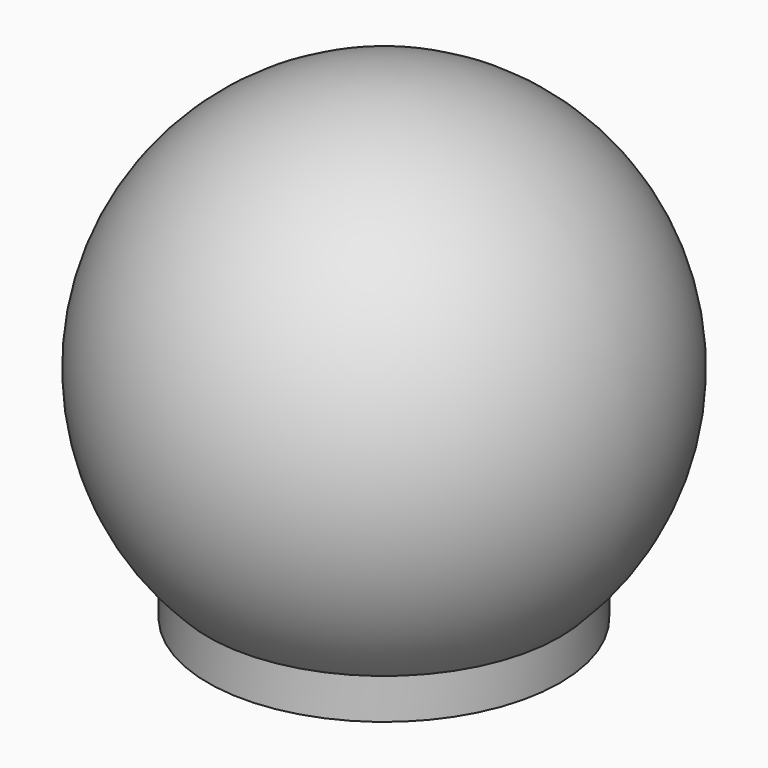
from build123d import *

# Parameters (mm, degrees)
F3_R      = 128.0515086977
F4_DEPTH  = 25.4
F5_R      = 35.56
F6_DEPTH  = 25.4
F7_R      = 28.702
F8_DEPTH  = 57.15
F10_DEPTH = 50.8
F11_R     = 5.079
F12_R     = 1.27
F13_R     = 2.54


# Not quite as in the source:
# - a fillet or chamfer is up to 0.001 mm smaller than in the source, because OpenCascade refuses the exact size


with BuildPart() as f1:
    # F0 (on Front) → F1 (revolve)
    with BuildSketch(Plane.XZ):
        with BuildLine():
            Line((0, 0), (0, -50.8))
            ThreePointArc((0, -50.8), (50.8, 0), (0, 50.8))
            Line((0, 50.8), (0, 0))
        make_face()
    revolve(axis=Axis((0, 0, 25.4), (0, 0, 1)))

    # F3 (on offset) → F4 (cut)
    with BuildSketch(Plane.XY.offset(-44.45)):
        with Locations((0, 3.5303835757)):
            Circle(F3_R)
    extrude(amount=-F4_DEPTH, mode=Mode.SUBTRACT)

    # F5 (on face) → F6 (join)
    with BuildSketch(Plane(origin=(0, 0, -44.45), x_dir=(1, 0, 0), z_dir=(0, 0, -1))):
        Circle(F5_R)
    extrude(amount=-F6_DEPTH)

    # F7 (on face) → F8 (cut)
    with BuildSketch(Plane(origin=(0, 0, -44.45), x_dir=(1, 0, 0), z_dir=(0, 0, -1))):
        Circle(F7_R)
    extrude(amount=-F8_DEPTH, mode=Mode.SUBTRACT)

    # F9 (on face) → F10 (cut)
    with BuildSketch(Plane(origin=(0, 0, -44.45), x_dir=(1, 0, 0), z_dir=(0, 0, -1))):
        with BuildLine():
            ThreePointArc((-5.08, 28.2488655347), (-2.5500848439, 28.588491938), (0, 28.702))
            Line((0, 28.702), (0, 32.0588655347))
            Line((0, 32.0588655347), (-5.08, 32.0588655347))
            Line((-5.08, 32.0588655347), (-5.08, 28.2488655347))
        make_face()
        with BuildLine():
            ThreePointArc((0, 28.702), (2.5500848439, 28.588491938), (5.08, 28.2488655347))
            Line((5.08, 28.2488655347), (5.08, 32.0588655347))
            Line((5.08, 32.0588655347), (0, 32.0588655347))
            Line((0, 32.0588655347), (0, 28.702))
        make_face()
        with BuildLine():
            Line((5.08, -32.0588655347), (5.08, -28.2488655347))
            ThreePointArc((5.08, -28.2488655347), (0, -28.702), (-5.08, -28.2488655347))
            Line((-5.08, -28.2488655347), (-5.08, -32.0588655347))
            Line((-5.08, -32.0588655347), (0, -32.0588655347))
            Line((0, -32.0588655347), (5.08, -32.0588655347))
        make_face()
    extrude(amount=-F10_DEPTH, mode=Mode.SUBTRACT)

    # F11 (radius 5.08 in the source; OpenCascade refuses exactly that, so slightly less here)
    f11_edges = [f1.edges().sort_by_distance(p)[0] for p in [
        (-5.08, -30.153866, 6.35),
        (5.08, -30.153866, 6.35),
        (5.08, 30.153866, 6.35),
        (-5.08, 30.153866, 6.35),
    ]]
    fillet(f11_edges, radius=F11_R)

    # F12
    f12_edges = [f1.edges().sort_by_distance(p)[0] for p in [
        (5.08, 28.248866, -21.5895),
        (5.08, 32.058866, -21.5895),
        (5.08, -32.058866, -21.5895),
        (5.08, -28.248866, -21.5895),
    ]]
    fillet(f12_edges, radius=F12_R)

    # F13
    f13_edges = [f1.edges().sort_by_distance(p)[0] for p in [
        (-28.702, 0, 12.7),
    ]]
    fillet(f13_edges, radius=F13_R)


solid = f1.part
